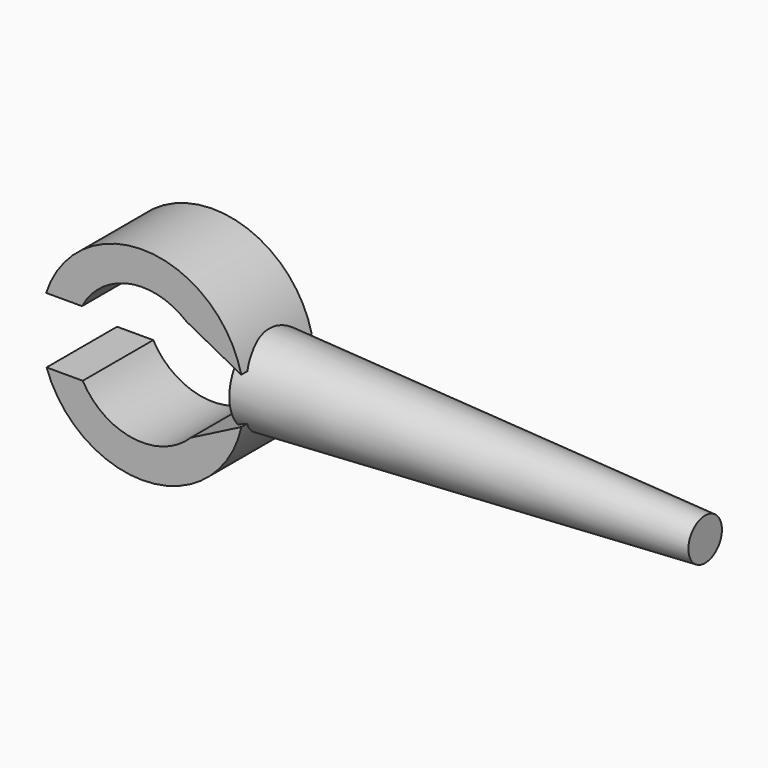
from build123d import *

# Parameters (mm, degrees)
F0_R     = 4.6089377224
F0_R_2   = 3.1053216927
F1_DEPTH = 4
F2_R     = 2
F3_DEPTH = 20
F3_TAPER = 3
F7_DEPTH = 5


# Not quite as in the source:
# - a feature of the source that left no trace in its solid (it failed there, or was rolled back) is left out


with BuildPart() as f1:
    # F0 (on Front) → F1 (new body)
    with BuildSketch(Plane.XZ):
        Circle(F0_R)
        Circle(F0_R_2, mode=Mode.SUBTRACT)
    extrude(amount=F1_DEPTH)

    # F6 (on offset) → F7 (cut)
    with BuildSketch(Plane.XZ.offset(5)):
        Polygon((1.1482916498, -2.7310699385), (6.4906934496, 0), (1.1892561404, 2.809761993), (1.1792272203, 1.4532563953), (1.1792272203, -1.5170100378), (1.1572674401, -1.5170100378), align=None)
        Polygon((1.1792272203, -1.5170100378), (1.1792272203, 1.4532563953), (1.1572674401, -1.5170100378), align=None)
        Polygon((1.1572674401, -1.5170100378), (1.1792272203, 1.4532563953), (-4.839008674, 1.4532563953), (-4.839008674, -1.5170100378), align=None)
    extrude(amount=-F7_DEPTH, mode=Mode.SUBTRACT)


with BuildPart() as f3:
    # F2 (on Right) → F3 (new body)
    with BuildSketch(Plane.YZ):
        Circle(F2_R)
    extrude(amount=F3_DEPTH, taper=F3_TAPER)


with BuildPart() as f3_1:
    # F4: moved
    add(f3.part.moved(Location((3.93674, -1.99355, 0))))


solid = Compound([f1.part, f3_1.part])
